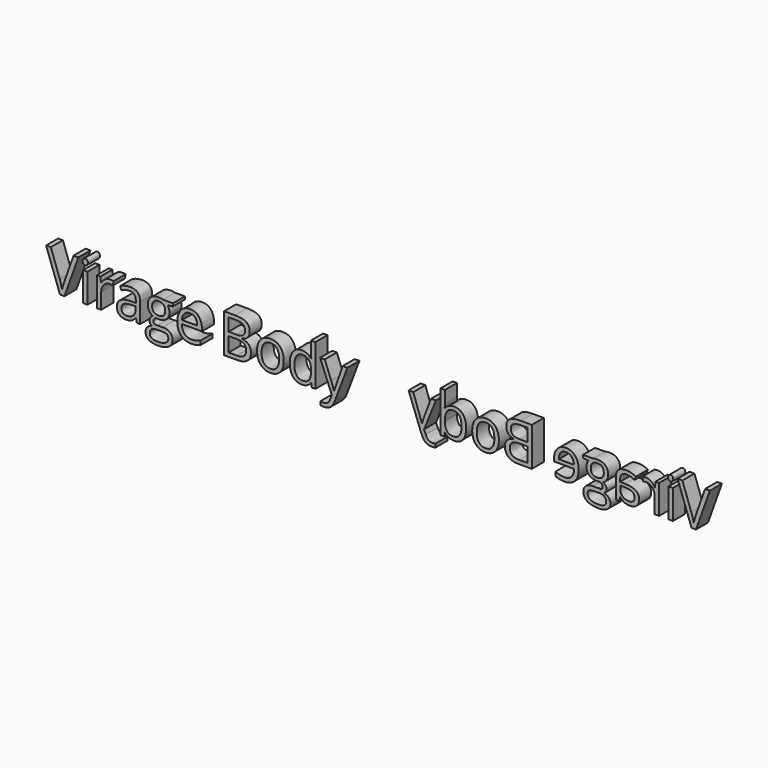
from build123d import *

# Parameters (mm, degrees)
F0_TEXT_SIZE = 7.2084248465
F1_DEPTH     = 2


# Not quite as in the source:
# - Text() gives the source's letters only with a copy of the font that has no kerning and outlines rounded to 1/6400 em; it was checked with that copy


with BuildPart() as f1:
    # F0 (on Front) → F1 (new body)
    with BuildSketch(Plane.XZ):
        with Locations((-44.0623518314, -2.6114352943)):
            Text('Virage Body', F0_TEXT_SIZE, font='Open Sans', text_align=(TextAlign.LEFT, TextAlign.BOTTOM))
    f1_solid = extrude(amount=F1_DEPTH)

    # F2: F1 across plane
    add(f1_solid.mirror(Plane.YZ))


solid = f1.part
